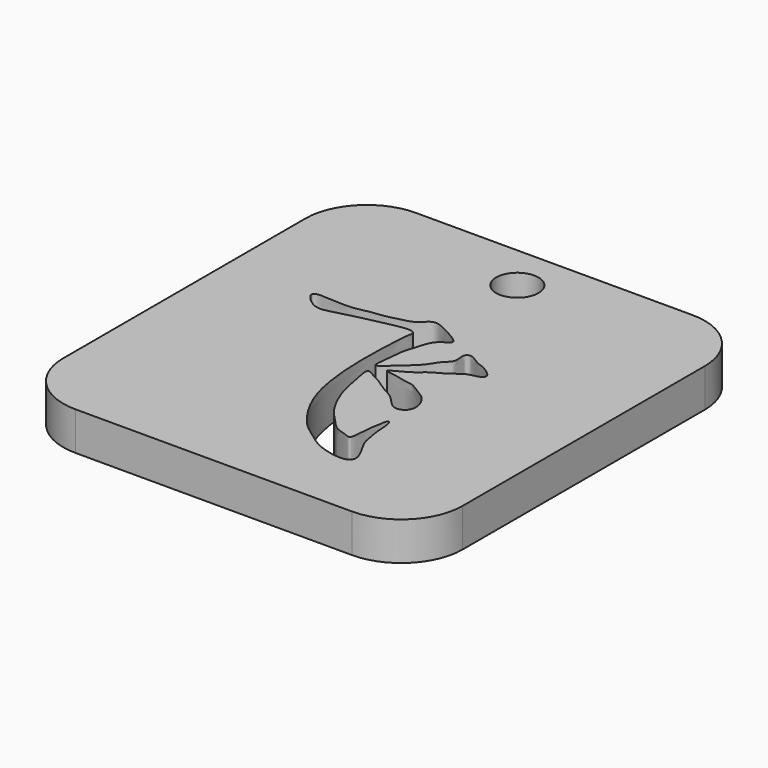
from build123d import *

# Parameters (mm, degrees)
F0_W     = 33.02
F0_H     = 35.1693436827
F0_R     = 1.75
F1_DEPTH = 3.175
F2_R     = 5.08


# Not quite as in the source:
# - a length typed as a fraction of an inch, garbled in the dataset ("3 / 203.2 mm" for 3/8 in), is restored


with BuildPart() as f1:
    # F0 (on Top) → F1 (new body)
    with BuildSketch(Plane.XY):
        with Locations((0, -2.2008972981)):
            Rectangle(F0_W, F0_H)
        with BuildLine():
            add(Edge.make_bspline(
                [(-9.4319959171, 2.4747848511), (-9.0111951678, 2.6528150769), (-6.5420286212, 2.2843658382), (-5.432982901, 2.7484741152), (-3.9375209961, 2.8183442215), (-3.2131964743, 3.1128875067), (-1.8361873772, 3.2734017236), (-1.1413564618, 4.4013090624), (-0.0351827282, 3.9756058559), (0.7223566506, 3.5580686681), (2.0094481861, 2.8144364971), (1.2478384799, 2.3968788401), (0.6208315977, 1.9063029494), (0.2979602617, 0.6697569649), (-0.0378670296, -0.2514498532), (-0.0752641301, -1.6449301018), (-0.3918011166, -3.322715038), (0.8058707871, -2.1505667224), (1.5811492633, -1.4959958557), (2.3727052585, -0.7670925996), (2.7977889425, 0.1526365687), (3.6624575003, 0.7251640991), (3.2814054516, 1.7715175462), (3.8877330296, 2.1447957131), (4.7823119921, 1.4134010523), (5.4199230373, 1.3258275708), (6.6462564571, 0.4707896574), (6.0658415697, -0.0377041391), (5.1485968811, -0.0707641585), (4.2533202076, -0.9475520476), (3.1286591677, -1.4033959186), (2.4063505352, -2.1808497402), (1.2915356323, -2.7054057367), (0.7007021955, -3.0782236496), (1.6862899937, -3.1421314569), (2.5860051488, -3.4229230494), (3.4303451538, -3.4547709277), (4.1078186324, -3.9873182091), (4.9943210875, -4.4133386079), (5.5370569458, -5.3474644367), (5.5875986737, -6.1834682659), (5.1163406773, -6.7506822602), (4.2218926973, -6.8211608476), (3.3781787786, -5.5954521122), (2.3133999422, -5.1792415472), (1.3021307027, -4.371368088), (0.5869458676, -4.0967072239), (-0.2415296419, -3.5185027211), (0.0254337467, -4.9113753534), (0.2187395242, -5.8836971725), (0.4683101692, -7.0350230724), (1.0155320882, -8.4521214167), (1.8053528665, -9.7190821874), (2.6112277996, -10.4930600568), (3.3788434637, -11.4194979787), (4.2697760077, -11.5722040285), (4.9688883551, -11.9711185553), (4.9778375148, -10.4666334437), (5.1379009584, -9.3517649157), (5.3492086846, -8.2679630049), (5.6879632618, -8.8590961582), (5.6623031639, -10.1297052588), (5.876347914, -10.8057701866), (5.9305841218, -11.4821127168), (6.1599895506, -12.0560992681), (6.6688984024, -12.8719323516), (7.1280114884, -13.8916699049), (6.5789762839, -14.4792894131), (5.1791795821, -14.313681002), (3.8360875816, -13.8860948059), (2.4671065748, -12.8458030116), (1.2905447565, -11.9839779965), (-0.3226479084, -9.4951800922), (-1.0855364921, -6.8356179824), (-1.4068296839, -3.3360864189), (-1.25297891, 0.205177533), (-1.195563285, 1.4257421625), (-0.9294454092, 2.5028732366), (-2.6008753034, 2.2670452306), (-3.8441473874, 1.9627525444), (-5.3215074167, 1.6725461409), (-7.111984113, 1.1668815666), (-8.3802630012, 0.8879654929), (-9.6476847595, 2.0619057335), (-9.5815524094, 2.4115112563), (-9.4319959171, 2.4747848511)],
                knots=[0, 0, 0, 0, 0.0189365441, 0.0325647847, 0.0459389493, 0.0563094801, 0.069400142, 0.0816330701, 0.0928373129, 0.1045467479, 0.1167177849, 0.1251372634, 0.1355819751, 0.1482481673, 0.1596511929, 0.173917805, 0.1858621643, 0.1976713601, 0.2101681736, 0.2217994419, 0.2333360267, 0.2442909078, 0.2552437853, 0.2630652769, 0.2746781275, 0.2847656921, 0.2973596713, 0.3052516113, 0.3161153975, 0.328803059, 0.3413267252, 0.3531913798, 0.3662803707, 0.3733970069, 0.3828668483, 0.3946680539, 0.404942397, 0.4153823096, 0.4267222172, 0.4384248333, 0.4486042055, 0.4578295412, 0.4676920592, 0.4811550001, 0.49363292, 0.5064260602, 0.5170695995, 0.525956932, 0.5373499186, 0.5495480112, 0.5618036181, 0.5760268553, 0.5899987178, 0.6022127091, 0.6145165705, 0.6255191126, 0.6336511724, 0.6459550345, 0.6595804739, 0.6695299103, 0.6764110238, 0.6896310371, 0.6995176936, 0.708669351, 0.7175795141, 0.7290607694, 0.7406954074, 0.7495164821, 0.7626924615, 0.7766167131, 0.7913326778, 0.8052631184, 0.8245970741, 0.8438200219, 0.8656449894, 0.8871576356, 0.9000551877, 0.909778626, 0.922877978, 0.9364896693, 0.9505395564, 0.966192803, 0.9791454377, 0.9932697765, 1, 1, 1, 1], degree=3))
        make_face(mode=Mode.SUBTRACT)
        with Locations((0, 11.5737745433)):
            Circle(F0_R, mode=Mode.SUBTRACT)
    extrude(amount=F1_DEPTH)

    # F2
    f2_edges = [f1.edges().sort_by_distance(p)[0] for p in [
        (-16.51, 15.383775, 1.5875),
        (16.51, 15.383775, 1.5875),
        (16.51, -19.785569, 1.5875),
        (-16.51, -19.785569, 1.5875),
    ]]
    fillet(f2_edges, radius=F2_R)


solid = f1.part
